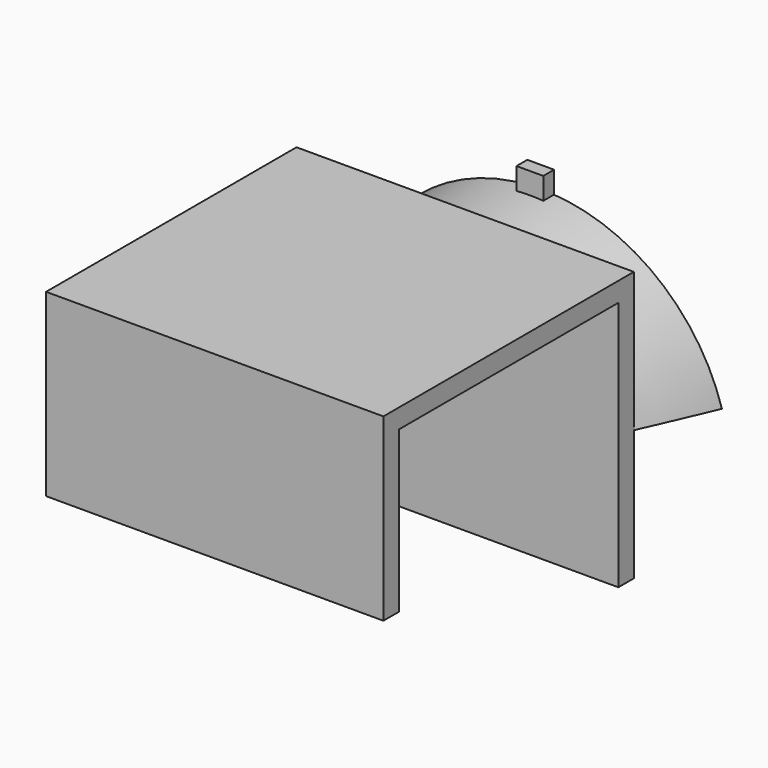
from build123d import *

# Parameters (mm, degrees)
F0_W                     = 4.3
F0_H                     = 55.7
F1_DEPTH                 = 75
F3_DEPTH                 = 21
DRAFT_F3_DRAFTED_ANGLE   = -4
F2_R                     = 6
DRAFT_F3_2_DRAFTED_ANGLE = -4
F5_DEPTH                 = 3
F4_W                     = 5.9588879347
F4_H                     = 15.3961649239


# Not quite as in the source:
# - an extrude with a draft is written as a straight extrude whose walls are then drafted


with BuildPart() as f1:
    # F0 (on Right) → F1 (new body)
    with BuildSketch(Plane.YZ):
        Polygon((-65.3, 60), (-69.6, 60), (-69.6, 20), (-65.3, 20), (-65.3, 55.7), align=None)
        Polygon((0, 60), (-65.3, 60), (-65.3, 55.7), (-4.3, 55.7), (0, 55.7), align=None)
        with Locations((-2.15, 27.85)):
            Rectangle(F0_W, F0_H)
    extrude(amount=F1_DEPTH)


with BuildPart() as f3_drafted:
    # F2 (on face) → F3 (new body)
    with BuildSketch(Plane(origin=(0, 0, 0), x_dir=(-1, 0, 0), z_dir=(0, 1, 0))):
        with BuildLine():
            ThreePointArc((-75, 29), (-37.5, 39), (0, 29))
            ThreePointArc((0, 29), (-37.5, 54), (-75, 29))
        make_face()
    extrude(amount=F3_DEPTH)

    # draft_F3_drafted
    draft_f3_drafted_walls = [f3_drafted.faces().sort_by_distance(p)[0] for p in [
        (37.5, 14, 39),
        (37.5, 14, 54),
    ]]
    draft(draft_f3_drafted_walls, neutral_plane=Plane(origin=(0, 0, 0), x_dir=(-1, 0, 0), z_dir=(0, 1, 0)), angle=DRAFT_F3_DRAFTED_ANGLE)


with BuildPart() as f1_1:
    add(f1.part)

    # join_F3_drafted: union F3_drafted
    add(f3_drafted.part)


with BuildPart() as f3_2_drafted:
    # F2 (on face) → F3, piece 2 (new body)
    with BuildSketch(Plane(origin=(0, 0, 0), x_dir=(-1, 0, 0), z_dir=(0, 1, 0))):
        with Locations((-37.5, 9)):
            Circle(F2_R)
    extrude(amount=F3_DEPTH)

    # draft_F3_2_drafted
    draft_f3_2_drafted_walls = [f3_2_drafted.faces().sort_by_distance(p)[0] for p in [
        (43.5, 14, 9),
    ]]
    draft(draft_f3_2_drafted_walls, neutral_plane=Plane(origin=(0, 0, 0), x_dir=(-1, 0, 0), z_dir=(0, 1, 0)), angle=DRAFT_F3_2_DRAFTED_ANGLE)


with BuildPart() as f1_2:
    add(f1_1.part)

    # join_F3_2_drafted: union F3_2_drafted
    add(f3_2_drafted.part)

    # F4 (on face) → F5, piece 2 (join)
    with BuildSketch(Plane(origin=(0, 21, 0), x_dir=(-1, 0, 0), z_dir=(0, 1, 0))):
        with Locations((-37.5, 13.375)):
            Rectangle(F4_W, F4_H)
    extrude(amount=-F5_DEPTH)


with BuildPart() as f5:
    # F4 (on face) → F5 (new body)
    with BuildSketch(Plane(origin=(0, 21, 0), x_dir=(-1, 0, 0), z_dir=(0, 1, 0))):
        with BuildLine():
            Line((-40.4794439673, 60.2324263691), (-40.4794439673, 55.3628856964))
            ThreePointArc((-40.4794439673, 55.3628856964), (-37.5, 55.4684630508), (-34.5205560327, 55.3628856964))
            Line((-34.5205560327, 55.3628856964), (-34.5205560327, 60.2324263691))
            Line((-34.5205560327, 60.2324263691), (-40.4794439673, 60.2324263691))
        make_face()
    extrude(amount=-F5_DEPTH)


solid = Compound([f1_2.part, f5.part])
